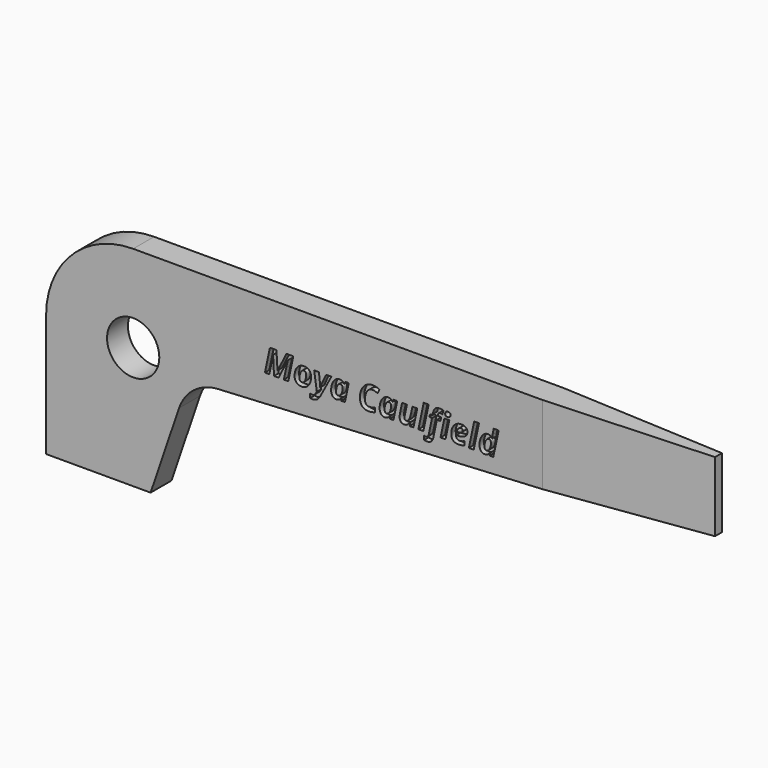
from build123d import *

# Parameters (mm, degrees)
F1_DEPTH     = 2.38125
F2_R         = 2.38125
F3_DEPTH     = 2.38225
F5_DEPTH     = 25.4
F6_TEXT_SIZE = 3.0148127634
F7_DEPTH     = 0.508


# Not quite as in the source:
# - Text() gives the source's letters only with a copy of the font that has no kerning and outlines rounded to 1/6400 em; it was checked with that copy


with BuildPart() as f1:
    # F0 (on Front) → F1 (new body)
    with BuildSketch(Plane.XZ):
        with BuildLine():
            Line((60.325, 19.05), (7.9375, 19.05))
            ThreePointArc((7.9375, 19.05), (2.3248399243, 16.7251600757), (0, 11.1125))
            Line((0, 11.1125), (0, 0))
            Line((0, 0), (9.525, 0))
            Line((9.525, 0), (12.1173647876, 7.6271664624))
            ThreePointArc((12.1173647876, 7.6271664624), (13.4786145605, 9.5135918491), (15.6631963617, 10.3130942181))
            Line((15.6631963617, 10.3130942181), (60.325, 12.7))
            Line((60.325, 12.7), (60.325, 19.05))
        make_face()
    extrude(amount=F1_DEPTH)

    # F2 (on face) → F3 (cut, through all)
    with BuildSketch(Plane.XZ.offset(2.38125)):
        with Locations((7.9375, 11.1125)):
            Circle(F2_R)
    extrude(amount=-F3_DEPTH, mode=Mode.SUBTRACT)

    # F4 (on face) → F5 (cut)
    with BuildSketch(Plane.XY.offset(19.05)):
        Polygon((60.325, 0), (45.24375, 0), (60.325, -0.79375), align=None)
        Polygon((60.325, -2.38125), (60.325, -1.5875), (45.24375, -2.38125), align=None)
    extrude(amount=-F5_DEPTH, mode=Mode.SUBTRACT)

    # F6 (on face) → F7 (cut)
    with BuildSketch(Plane.XZ.offset(2.38125)):
        with Locations((19.8662709445, 13.0193959922)):
            Text('Moya Caulfield', F6_TEXT_SIZE, font='Open Sans', font_style=FontStyle.BOLDITALIC, text_align=(TextAlign.LEFT, TextAlign.BOTTOM))
    extrude(amount=-F7_DEPTH, mode=Mode.SUBTRACT)


solid = f1.part
